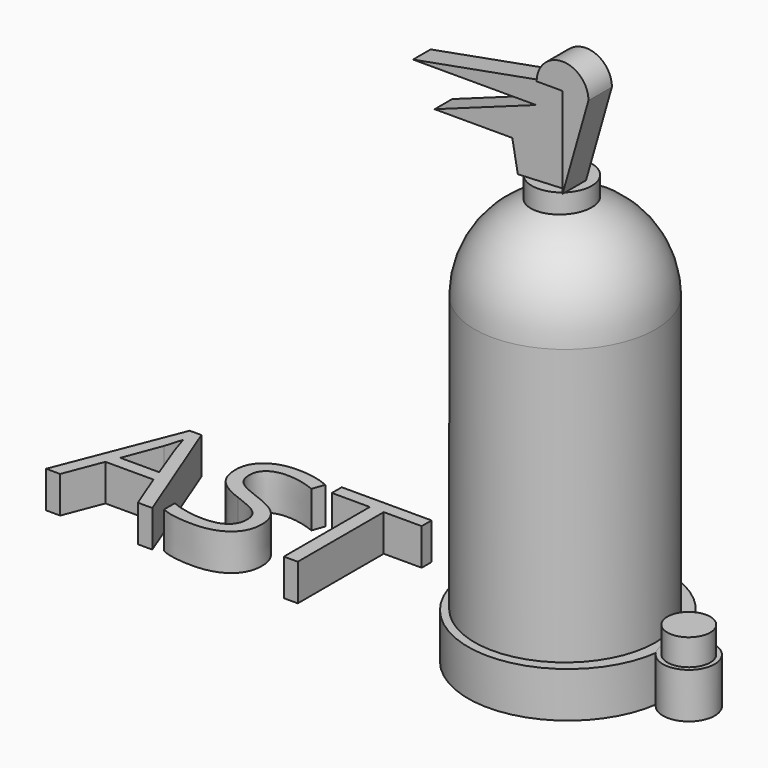
from build123d import *

# Parameters (mm, degrees)
F0_R          = 15.6945956087
F1_DEPTH      = 55.626
F4_R          = 5.1884963377
F5_DEPTH      = 73.914
F7_DEPTH      = 5.08
F9_DEPTH      = 3.81
F10_R         = 3.717292365
F11_DEPTH     = 12.446
F13_R         = 17.3248606213
F14_DEPTH     = 7.874
F15_R         = 4.4901085292
F16_DEPTH     = 7.874
F17_TEXT_SIZE = 29.0858727466
F18_DEPTH     = 6.35


# Not quite as in the source:
# - the program builds the solid bodies; features that only make, move or delete a surface that nothing else refers to are left out
# - Text() gives the source's letters only with a copy of the font that has no kerning and outlines rounded to 1/6400 em; it was checked with that copy


with BuildPart() as f1:
    # F0 (on Top) → F1 (new body)
    with BuildSketch(Plane.XY):
        with Locations((23.312266916, 0)):
            Circle(F0_R)
    extrude(amount=F1_DEPTH)

    # F2 (on Front) → F3 (revolve)
    with BuildSketch(Plane.XZ):
        with BuildLine():
            ThreePointArc((23.312266916, 71.3205956087), (12.2145119332, 66.7237549829), (7.6176713074, 55.626))
            Line((7.6176713074, 55.626), (23.312266916, 55.626))
            Line((23.312266916, 55.626), (23.312266916, 71.3205956087))
        make_face()
    revolve(axis=Axis((23.312266916, 0, 63.4732978043), (0, 0, 1)))

    # F4 (on Top) → F5 (join)
    with BuildSketch(Plane.XY):
        with Locations((22.7366555482, 0)):
            Circle(F4_R)
    extrude(amount=F5_DEPTH)


with BuildPart() as f7:
    # F6 (on Front) → F7 (new body)
    with BuildSketch(Plane.XZ):
        with BuildLine():
            Line((26.9279368222, 90.1338011026), (26.9279368222, 74.4258314371))
            Line((26.9279368222, 74.4258314371), (31.4159262925, 90.1338011026))
            ThreePointArc((31.4159262925, 90.1338011026), (26.9279368222, 94.621790573), (22.4399473518, 90.1338011026))
            Line((22.4399473518, 90.1338011026), (26.9279368222, 90.1338011026))
        make_face()
    extrude(amount=F7_DEPTH)


with BuildPart() as f9:
    # F8 (on Front) → F9 (new body)
    with BuildSketch(Plane.XZ):
        Polygon((18.1625332805, 74.0592666), (26.1799450964, 74.4258314371), (26.1799450964, 89.7597894073), (22.4399510771, 89.7597894073), (0, 85.645802319), (21.3179551065, 85.645802319), (3.7399933208, 79.2878195643), (17.2039661556, 79.2878195643), align=None)
    extrude(amount=F9_DEPTH)


with BuildPart() as f11:
    # F10 (on Top) → F11 (new body)
    with BuildSketch(Plane.XY):
        with Locations((44.7393618524, 0)):
            Circle(F10_R)
    extrude(amount=F11_DEPTH)


with BuildPart() as f14:
    # F13 (on Top) → F14 (new body)
    with BuildSketch(Plane.XY):
        with Locations((23.7975232303, 0)):
            Circle(F13_R)
    extrude(amount=F14_DEPTH)


with BuildPart() as f16:
    # F15 (on Top) → F16 (new body)
    with BuildSketch(Plane.XY):
        with Locations((44.7393469512, 0)):
            Circle(F15_R)
    extrude(amount=F16_DEPTH)


with BuildPart() as f18:
    # F17 (on Top) → F18 (new body)
    with BuildSketch(Plane.XY):
        with Locations((-59.0178668499, -9.5190182328)):
            Text('AST', F17_TEXT_SIZE, font='Open Sans', text_align=(TextAlign.LEFT, TextAlign.BOTTOM))
    extrude(amount=F18_DEPTH)


solid = Compound([f1.part, f7.part, f9.part, f11.part, f14.part, f16.part, f18.part])
